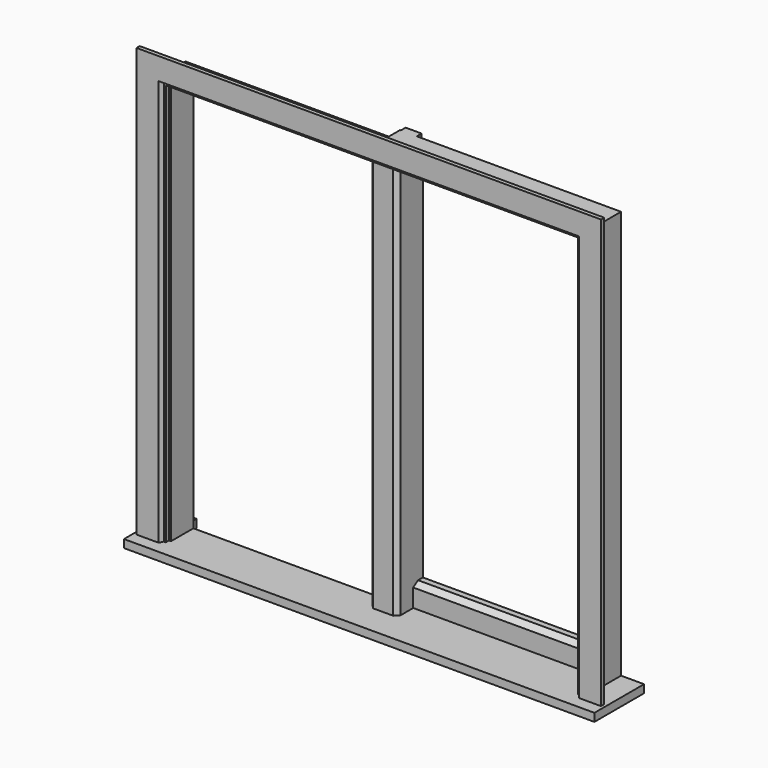
from build123d import *

# Parameters (mm, degrees)
F0_W      = 20
F0_H      = 105
F1_DEPTH  = 1000
F2_W      = 1060
F2_H      = 105
F3_DEPTH  = 20
F4_W      = 1175
F4_H      = 155
F5_DEPTH  = 20
F7_W      = 508
F7_H      = 35
F8_DEPTH  = 1040
F9_DEPTH  = 475
F11_DEPTH = 10
F13_DEPTH = 1020
F15_DEPTH = 10
F16_SIZE2 = 9.99999
F16_SIZE  = 4.99999


# Not quite as in the source:
# - a fillet or chamfer is up to 0.001 mm smaller than in the source, because OpenCascade refuses the exact size


with BuildPart() as f1:
    # F0 (on Top) → F1 (new body)
    with BuildSketch(Plane.XY):
        with Locations((-520, -52.5)):
            Rectangle(F0_W, F0_H)
    extrude(amount=F1_DEPTH)



with BuildPart() as f1b:
    # F0 (on Top) → F1, piece 2 (new body)
    with BuildSketch(Plane.XY):
        with Locations((520, -52.5)):
            Rectangle(F0_W, F0_H)
    extrude(amount=F1_DEPTH)


with BuildPart() as f1c:
    # F0 (on Top) → F1, piece 3 (new body)
    with BuildSketch(Plane.XY):
        Polygon((35, 0), (0, 0), (-35, 0), (-35, -70), (-25, -80), (25, -80), (35, -70), align=None)
    extrude(amount=F1_DEPTH)


with BuildPart() as f1_1:
    add(f1.part)

    add(f1b.part)  # F3 merges F1b

    add(f1c.part)  # F3 merges F1c
    # F2 (on face) → F3 (join)
    with BuildSketch(Plane.XY.offset(1000)):
        with Locations((0, -52.5)):
            Rectangle(F2_W, F2_H)
    extrude(amount=F3_DEPTH)

    # F4 (on face) → F5 (join)
    with BuildSketch(Plane(origin=(0, 0, 0), x_dir=(1, 0, 0), z_dir=(0, 0, -1))):
        with Locations((0, 77.5)):
            Rectangle(F4_W, F4_H)
    extrude(amount=F5_DEPTH)

    # F7 (on face) → F8 (cut, through all)
    with BuildSketch(Plane.XY.offset(1020)):
        with Locations((-276, -17.5)):
            Rectangle(F7_W, F7_H)
    extrude(amount=-F8_DEPTH, mode=Mode.SUBTRACT)

    # F6 (on face) → F9 (join, through all)
    with BuildSketch(Plane(origin=(510, 0, 0), x_dir=(0, -1, 0), z_dir=(-1, 0, 0))):
        Polygon((0, 55), (0, 0), (30, 0), (30, 45), (15, 55), align=None)
    extrude(amount=F9_DEPTH)

    # F10 (on face) → F11 (join)
    with BuildSketch(Plane.XZ.offset(105)):
        Polygon((515, 1005), (515, 0), (535, 0), (535, 1025), (-535, 1025), (-535, 0), (-515, 0), (-515, 1005), align=None)
    extrude(amount=F11_DEPTH)

    # F12 (on Top) → F13 (join, through all)
    with BuildSketch(Plane.XY):
        Polygon((-20, 0), (0, 0), (20, 0), (20, 15), (-20, 15), align=None)
    extrude(amount=F13_DEPTH)

    # F14 (on face) → F15 (join)
    with BuildSketch(Plane.XZ.offset(115)):
        Polygon((520, 1010), (520, 0), (580, 0), (580, 1070), (-580, 1070), (-580, 0), (-520, 0), (-520, 1010), align=None)
    extrude(amount=F15_DEPTH)

    # F16 (size 5 and 10 in the source; OpenCascade refuses exactly that, so slightly less here)
    f16_edges = [f1_1.edges().sort_by_distance(p)[0] for p in [
        (-520, -125, 505),
        (0, -125, 1010),
        (520, -125, 505),
    ]]
    f16_side = f1_1.faces().sort_by_distance((535.781318, -125, 505))[0]
    chamfer(f16_edges, length=F16_SIZE, length2=F16_SIZE2, reference=f16_side)


solid = f1_1.part
